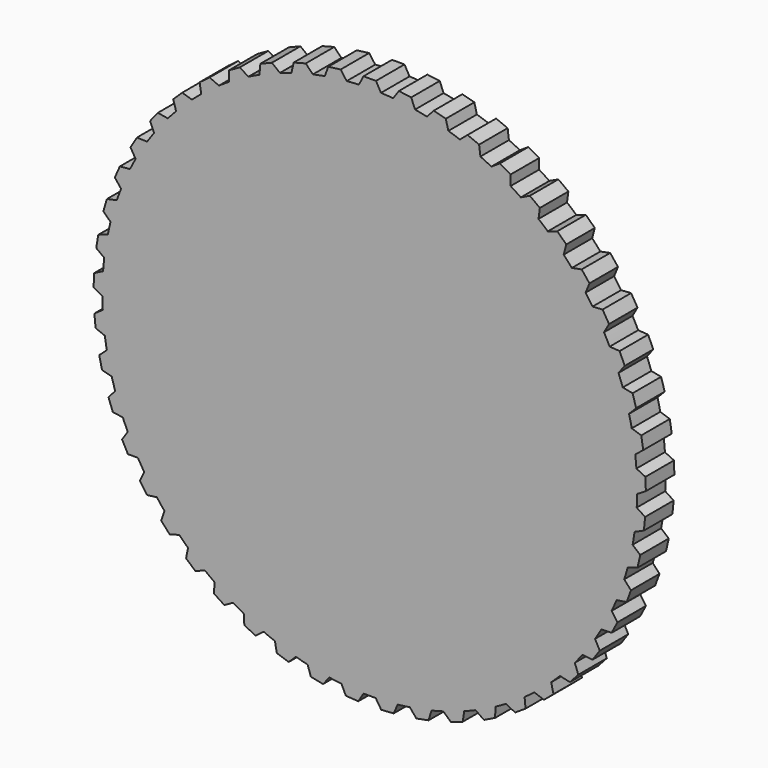
from build123d import *

# Parameters (mm, degrees)
F1_DEPTH = 12.7


# Not quite as in the source:
# - the program builds the solid bodies; features that only make, move or delete a surface that nothing else refers to are left out


with BuildPart() as f1:
    # F0 (on Front) → F1 (new body, symmetric)
    with BuildSketch(Plane.XZ):
        with BuildLine():
            Line((-29.5596303567, 194.4987351337), (-32.023844694, 187.7890395391))
            ThreePointArc((-32.023844694, 187.7890395391), (-36.2909460261, 187.0112756936), (-40.539233927, 186.1365641474))
            Line((-40.539233927, 186.1365641474), (-45.5896410678, 191.3768908273))
            Line((-45.5896410678, 191.3768908273), (-54.1888924002, 189.1219015764))
            Line((-54.1888924002, 189.1219015764), (-55.7748587434, 182.1521757546))
            ThreePointArc((-55.7748587434, 182.1521757546), (-59.9074689996, 180.8351325325), (-64.0090228858, 179.4243433573))
            Line((-64.0090228858, 179.4243433573), (-69.6880843559, 183.9758152971))
            Line((-69.6880843559, 183.9758152971), (-77.9283743287, 180.6396916238))
            Line((-77.9283743287, 180.6396916238), (-78.6100511543, 173.5243782802))
            Line((-78.6100511543, 173.5243782802), (-86.4277854583, 169.7659798098))
            Line((-86.4277854583, 169.7659798098), (-92.6422512254, 173.553861966))
            Line((-92.6422512254, 173.553861966), (-100.3882745051, 169.1913829287))
            Line((-100.3882745051, 169.1913829287), (-100.1544686985, 162.0473153117))
            ThreePointArc((-100.1544686985, 162.0473153117), (-103.8178473197, 159.7250906336), (-107.4274061831, 157.3200635672))
            Line((-107.4274061831, 157.3200635672), (-114.0752348911, 160.2821590196))
            Line((-114.0752348911, 160.2821590196), (-121.1998019895, 154.9649564035))
            Line((-121.1998019895, 154.9649564035), (-120.0543526356, 147.9094399058))
            ThreePointArc((-120.0543526356, 147.9094399058), (-123.3906954684, 145.1378181999), (-126.6630718683, 142.2909562301))
            Line((-126.6630718683, 142.2909562301), (-133.6351063536, 144.3786274533))
            Line((-133.6351063536, 144.3786274533), (-140.021232076, 138.1940095784))
            Line((-140.021232076, 138.1940095784), (-137.9829474215, 131.3428955858))
            ThreePointArc((-137.9829474215, 131.3428955858), (-140.9374718087, 128.167386804), (-143.8189334152, 124.9254353256))
            Line((-143.8189334152, 124.9254353256), (-151.0006930643, 126.1044028158))
            Line((-151.0006930643, 126.1044028158), (-156.5435174029, 119.1539209366))
            Line((-156.5435174029, 119.1539209366), (-153.6458660255, 112.6197045515))
            ThreePointArc((-153.6458660255, 112.6197045515), (-156.1700587584, 109.0924504602), (-158.6132920516, 105.5086422269))
            Line((-158.6132920516, 105.5086422269), (-165.8868525696, 105.7595473704))
            Line((-165.8868525696, 105.7595473704), (-170.4953625019, 98.1573282073))
            Line((-170.4953625019, 98.1573282073), (-166.7859237571, 92.047301082))
            ThreePointArc((-166.7859237571, 92.047301082), (-168.8383376608, 88.2262190958), (-170.8032248176, 84.3594001397))
            Line((-170.8032248176, 84.3594001397), (-178.0491545419, 83.678123081))
            Line((-178.0491545419, 83.678123081), (-181.6476784622, 75.5489948624))
            Line((-181.6476784622, 75.5489948624), (-177.1873612317, 69.9634834736))
            ThreePointArc((-177.1873612317, 69.9634834736), (-178.7342957266, 65.911315653), (-180.1885733541, 61.8249790344))
            Line((-180.1885733541, 61.8249790344), (-187.287894319, 60.2227063241))
            Line((-187.287894319, 60.2227063241), (-189.8173445641, 51.7001491106))
            Line((-189.8173445641, 51.7001491106), (-184.6793871334, 46.7308674007))
            ThreePointArc((-184.6793871334, 46.7308674007), (-185.695441598, 42.5141502294), (-186.6152304978, 38.2753934826))
            Line((-186.6152304978, 38.2753934826), (-193.4513720492, 35.7784343943))
            Line((-193.4513720492, 35.7784343943), (-194.8702151161, 27.0023883397))
            Line((-194.8702151161, 27.0023883397), (-189.1389826042, 22.7309317771))
            ThreePointArc((-189.1389826042, 22.7309317771), (-189.6074734522, 18.4189036344), (-189.977670716, 14.0973270281))
            Line((-189.977670716, 14.0973270281), (-196.4383835987, 10.7466815608))
            Line((-196.4383835987, 10.7466815608), (-196.7233221233, 1.8612490988))
            Line((-196.7233221233, 1.8612490988), (-190.4929212096, -1.6422451179))
            ThreePointArc((-190.4929212096, -1.6422451179), (-190.4061558342, -5.9787808491), (-190.2206828332, -10.3122171465))
            Line((-190.2206828332, -10.3122171465), (-196.1998823203, -14.4615314867))
            Line((-196.1998823203, -14.4615314867), (-195.34623762, -23.3104518008))
            Line((-195.34623762, -23.3104518008), (-188.7189713152, -25.9884563935))
            ThreePointArc((-188.7189713152, -25.9884563935), (-188.0783744015, -30.2782939163), (-187.3402765972, -34.5524350007))
            Line((-187.3402765972, -34.5524350007), (-192.7397843984, -39.4322865871))
            Line((-192.7397843984, -39.4322865871), (-190.7615732955, -48.0993957264))
            Line((-190.7615732955, -48.0993957264), (-183.8462611293, -49.9079379336))
            ThreePointArc((-183.8462611293, -49.9079379336), (-182.6623512609, -54.0806382345), (-181.3837481988, -58.2253028274))
            Line((-181.3837481988, -58.2253028274), (-186.1149045453, -63.7555646318))
            Line((-186.1149045453, -63.7555646318), (-183.0446092115, -72.0985489038))
            Line((-183.0446092115, -72.0985489038), (-175.9548004183, -73.0079325125))
            ThreePointArc((-175.9548004183, -73.0079325125), (-174.2470173625, -76.994979968), (-172.4489036696, -80.9421127914))
            Line((-172.4489036696, -80.9421127914), (-176.434023105, -87.0319780679))
            Line((-176.434023105, -87.0319780679), (-172.3220577048, -94.9138459016))
            Line((-172.3220577048, -94.9138459016), (-165.174166749, -94.9091388581))
            ThreePointArc((-165.174166749, -94.9091388581), (-162.9705522563, -98.6450662591), (-160.6824529098, -102.3298555012))
            Line((-160.6824529098, -102.3298555012), (-163.8560998831, -108.8793288303))
            Line((-163.8560998831, -108.8793288303), (-158.7699827746, -116.1706601737))
            Line((-158.7699827746, -116.1706601737), (-151.6813778281, -115.2519397675))
            ThreePointArc((-151.6813778281, -115.2519397675), (-149.0181151877, -118.6754032894), (-146.2776007155, -122.0373448127))
            Line((-146.2776007155, -122.0373448127), (-148.5876640311, -128.9388840234))
            Line((-148.5876640311, -128.9388840234), (-142.6109091167, -135.5199554174))
            Line((-142.6109091167, -135.5199554174), (-135.6979848768, -133.7023070122))
            ThreePointArc((-135.6979848768, -133.7023070122), (-132.6188047875, -136.7570934787), (-129.4708743615, -139.7409842962))
            Line((-129.4708743615, -139.7409842962), (-130.8794228437, -146.8812663056))
            Line((-130.8794228437, -146.8812663056), (-124.1101682738, -152.6440167399))
            Line((-124.1101682738, -152.6440167399), (-117.4864347653, -149.9572860722))
            ThreePointArc((-117.4864347653, -149.9572860722), (-114.0418972791, -152.5932359739), (-110.5382398299, -155.150080681))
            Line((-110.5382398299, -155.150080681), (-111.0221451516, -162.4118622557))
            Line((-111.0221451516, -162.4118622557), (-103.5715418991, -167.2616675275))
            Line((-103.5715418991, -167.2616675275), (-97.3457606431, -163.7499706406))
            ThreePointArc((-97.3457606431, -163.7499706406), (-93.5924249703, -165.923801753), (-89.7905704563, -168.0116170303))
            Line((-89.7905704563, -168.0116170303), (-89.3418869054, -175.2756599178))
            Line((-89.3418869054, -175.2756599178), (-81.3322736698, -179.1328863585))
            Line((-81.3322736698, -179.1328863585), (-75.6066718225, -174.8538852183))
            ThreePointArc((-75.6066718225, -174.8538852183), (-71.606167631, -176.5299032946), (-67.5685423982, -178.1144072729))
            Line((-67.5685423982, -178.1144072729), (-66.1946373462, -185.2614360897))
            Line((-66.1946373462, -185.2614360897), (-57.7575317553, -188.062748148))
            Line((-57.7575317553, -188.062748148), (-52.6261235407, -183.0867038348))
            ThreePointArc((-52.6261235407, -183.0867038348), (-48.4441389988, -184.2373887045), (-44.2370407419, -185.2925638724))
            Line((-44.2370407419, -185.2925638724), (-41.9604736719, -192.2052246029))
            Line((-41.9604736719, -192.2052246029), (-33.2344127662, -193.9046248121))
            Line((-33.2344127662, -193.9046248121), (-28.7814557653, -188.313243836))
            ThreePointArc((-28.7814557653, -188.313243836), (-24.4866589436, -188.9197012854), (-20.1791680997, -189.4282216957))
            Line((-20.1791680997, -189.4282216957), (-17.0373201799, -195.9930086419))
            Line((-17.0373201799, -195.9930086419), (-8.1655856384, -196.5625928976))
            Line((-8.1655856384, -196.5625928976), (-4.464197282, -190.4476855796))
            ThreePointArc((-4.464197282, -190.4476855796), (-0.1271086255, -190.4999575942), (4.2100459249, -190.4534733559))
            Line((4.2100459249, -190.4534733559), (8.1655856384, -196.5625928976))
            Line((8.1655856384, -196.5625928976), (17.0373201799, -195.9930086419))
            Line((17.0373201799, -195.9930086419), (19.9263631973, -189.4549815912))
            ThreePointArc((19.9263631973, -189.4549815912), (24.2345288127, -188.9522098659), (28.5301311117, -188.3514842489))
            Line((28.5301311117, -188.3514842489), (33.2344127662, -193.9046248121))
            Line((33.2344127662, -193.9046248121), (41.9604736719, -192.2052246029))
            Line((41.9604736719, -192.2052246029), (43.9897333437, -185.3514320429))
            ThreePointArc((43.9897333437, -185.3514320429), (48.1982359579, -184.3018720755), (52.3817523345, -183.1567689777))
            Line((52.3817523345, -183.1567689777), (57.7575317553, -188.062748148))
            Line((57.7575317553, -188.062748148), (66.1946373462, -185.2614360897))
            Line((66.1946373462, -185.2614360897), (67.3307932849, -178.2044171047))
            ThreePointArc((67.3307932849, -178.2044171047), (71.3705294011, -176.625302641), (75.3732666321, -174.9546246237))
            Line((75.3732666321, -174.9546246237), (81.3322736698, -179.1328863585))
            Line((81.3322736698, -179.1328863585), (89.3418869054, -175.2756599178))
            Line((89.3418869054, -175.2756599178), (89.5662834617, -168.1312905644))
            ThreePointArc((89.5662834617, -168.1312905644), (93.3709207247, -166.0485506201), (97.1271539754, -163.8797301701))
            Line((97.1271539754, -163.8797301701), (103.5715418991, -167.2616675275))
            Line((103.5715418991, -167.2616675275), (111.0221451516, -162.4118622557))
            Line((111.0221451516, -162.4118622557), (110.3310977403, -155.2974528813))
            ThreePointArc((110.3310977403, -155.2974528813), (113.8381641113, -152.7452859887), (117.2862161357, -150.1139350779))
            Line((117.2862161357, -150.1139350779), (124.1101682738, -152.6440167399))
            Line((124.1101682738, -152.6440167399), (130.8794228437, -146.8812663056))
            Line((130.8794228437, -146.8812663056), (129.2842784443, -139.9136353153))
            ThreePointArc((129.2842784443, -139.9136353153), (132.4361879905, -136.9339479842), (135.5194418695, -133.8832733219))
            Line((135.5194418695, -133.8832733219), (142.6109091167, -135.5199554174))
            Line((142.6109091167, -135.5199554174), (148.5876640311, -128.9388840234))
            Line((148.5876640311, -128.9388840234), (146.1146148705, -122.2324397255))
            ThreePointArc((146.1146148705, -122.2324397255), (148.8596133243, -118.8741583396), (151.5274421145, -115.4542519192))
            Line((151.5274421145, -115.4542519192), (158.7699827746, -116.1706601737))
            Line((158.7699827746, -116.1706601737), (163.8560998831, -108.8793288303))
            Line((163.8560998831, -108.8793288303), (160.5457533601, -102.5441908547))
            ThreePointArc((160.5457533601, -102.5441908547), (162.8387679227, -98.8624583015), (165.0473659492, -95.129474892))
            Line((165.0473659492, -95.129474892), (172.3220577048, -94.9138459016))
            Line((172.3220577048, -94.9138459016), (176.434023105, -87.0319780679))
            Line((176.434023105, -87.0319780679), (172.340735018, -81.1721692051))
            ThreePointArc((172.340735018, -81.1721692051), (174.1441144538, -77.2274394313), (175.857216598, -73.2426745171))
            Line((175.857216598, -73.2426745171), (183.0446092115, -72.0985489038))
            Line((183.0446092115, -72.0985489038), (186.1149045453, -63.7555646318))
            Line((186.1149045453, -63.7555646318), (181.3058865715, -58.4673027813))
            ThreePointArc((181.3058865715, -58.4673027813), (182.59001944, -54.3243481407), (183.779496612, -50.1532314515))
            Line((183.779496612, -50.1532314515), (190.7615732955, -48.0993957264))
            Line((190.7615732955, -48.0993957264), (192.7397843984, -39.4322865871))
            Line((192.7397843984, -39.4322865871), (187.29400048, -34.8024048622))
            ThreePointArc((187.29400048, -34.8024048622), (188.0378013549, -30.5292525555), (188.6841223726, -26.240273712))
            Line((188.6841223726, -26.240273712), (195.34623762, -23.3104518008))
            Line((195.34623762, -23.3104518008), (196.1998823203, -14.4615314867))
            Line((196.1998823203, -14.4615314867), (190.2067520787, -10.5660524175))
            ThreePointArc((190.2067520787, -10.5660524175), (190.3980077703, -6.2328674874), (190.4905600603, -1.8964514036))
            Line((190.4905600603, -1.8964514036), (196.7233221233, 1.8612490988))
            Line((196.7233221233, 1.8612490988), (196.4383835987, 10.7466815608))
            Line((196.4383835987, 10.7466815608), (189.9963140667, 13.8437943159))
            ThreePointArc((189.9963140667, 13.8437943159), (189.6318841618, 18.1658610926), (189.1691480181, 22.4785105844))
            Line((189.1691480181, 22.4785105844), (194.8702151161, 27.0023883397))
            Line((194.8702151161, 27.0023883397), (193.4513720492, 35.7784343943))
            Line((193.4513720492, 35.7784343943), (186.6661418305, 38.0263263293))
            ThreePointArc((186.6661418305, 38.0263263293), (185.7520102581, 42.2663067356), (184.7415837954, 46.4843760501))
            Line((184.7415837954, 46.4843760501), (189.8173445641, 51.7001491106))
            Line((189.8173445641, 51.7001491106), (187.287894319, 60.2227063241))
            Line((187.287894319, 60.2227063241), (180.2709167062, 61.5844671157))
            Line((180.2709167062, 61.5844671157), (177.2805678742, 69.7269693462))
            Line((177.2805678742, 69.7269693462), (181.6476784622, 75.5489948624))
            Line((181.6476784622, 75.5489948624), (178.0491545419, 83.678123081))
            Line((178.0491545419, 83.678123081), (170.9156481133, 84.1313926546))
            ThreePointArc((170.9156481133, 84.1313926546), (168.9559228734, 88.0008302574), (166.9086099297, 91.8246477332))
            Line((166.9086099297, 91.8246477332), (170.4953625019, 98.1573282073))
            Line((170.4953625019, 98.1573282073), (165.8868525696, 105.7595473704))
            Line((165.8868525696, 105.7595473704), (158.7539493037, 105.2968830521))
            ThreePointArc((158.7539493037, 105.2968830521), (156.315500683, 108.8839485243), (153.7960172246, 112.4145679432))
            Line((153.7960172246, 112.4145679432), (156.5435174029, 119.1539209366))
            Line((156.5435174029, 119.1539209366), (151.0006930643, 126.1044028158))
            Line((151.0006930643, 126.1044028158), (143.9855150355, 124.7334015409))
            ThreePointArc((143.9855150355, 124.7334015409), (141.1083822928, 127.9791953667), (138.1580981686, 131.1586440554))
            Line((138.1580981686, 131.1586440554), (140.021232076, 138.1940095784))
            Line((140.021232076, 138.1940095784), (133.6351063536, 144.3786274533))
            Line((133.6351063536, 144.3786274533), (126.8528425911, 142.1218010249))
            ThreePointArc((126.8528425911, 142.1218010249), (123.5842681666, 144.9730273593), (120.2516269602, 147.7490988582))
            Line((120.2516269602, 147.7490988582), (121.1998019895, 154.9649564035))
            Line((121.1998019895, 154.9649564035), (114.0752348911, 160.2821590196))
            Line((114.0752348911, 160.2821590196), (107.6372499784, 157.1765644652))
            ThreePointArc((107.6372499784, 157.1765644652), (104.0309037738, 159.5864062507), (100.3706273617, 161.9135175426))
            Line((100.3706273617, 161.9135175426), (100.3882745051, 169.1913829287))
            Line((100.3882745051, 169.1913829287), (92.6422512254, 173.553861966))
            Line((92.6422512254, 173.553861966), (86.6542566968, 169.6504930624))
            ThreePointArc((86.6542566968, 169.6504930624), (82.7693548171, 171.5793807634), (78.8415448368, 173.4193207453))
            Line((78.8415448368, 173.4193207453), (77.9283743287, 180.6396916238))
            Line((77.9283743287, 180.6396916238), (69.6880843559, 183.9758152971))
            Line((69.6880843559, 183.9758152971), (64.248402916, 179.3387652538))
            ThreePointArc((64.248402916, 179.3387652538), (60.1487353426, 180.7550265876), (56.0178863254, 182.0775834957))
            Line((56.0178863254, 182.0775834957), (54.1888924002, 189.1219015764))
            Line((54.1888924002, 189.1219015764), (45.5896410678, 191.3768908273))
            Line((45.5896410678, 191.3768908273), (40.7875921355, 186.0822998777))
            ThreePointArc((40.7875921355, 186.0822998777), (36.5404752966, 186.9626798725), (32.2744156692, 187.746137359))
            Line((32.2744156692, 187.746137359), (29.5596303567, 194.4987351337))
            Line((29.5596303567, 194.4987351337), (20.7426171339, 195.6355631011))
            Line((20.7426171339, 195.6355631011), (16.6570502198, 189.7703682822))
            ThreePointArc((16.6570502198, 189.7703682822), (12.3322216566, 190.1004111227), (8.001, 190.3319048373))
            Line((8.001, 190.3319048373), (4.445, 196.6819048373))
            Line((4.445, 196.6819048373), (-4.445, 196.6819048373))
            Line((-4.445, 196.6819048373), (-7.747, 190.342412486))
            ThreePointArc((-7.747, 190.342412486), (-12.0785267222, 190.1166988779), (-16.403791868, 189.7924277002))
            Line((-16.403791868, 189.7924277002), (-20.7426171339, 195.6355631011))
            Line((-20.7426171339, 195.6355631011), (-29.5596303567, 194.4987351337))
        make_face()
    extrude(amount=F1_DEPTH, both=True)


solid = f1.part
